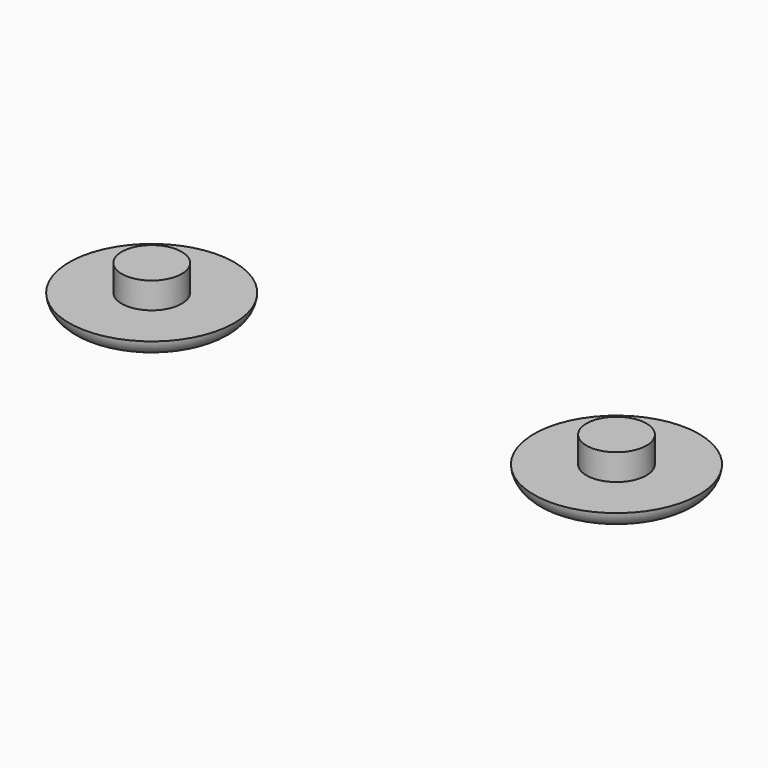
from build123d import *

# Parameters (mm, degrees)
F0_R     = 11
F1_DEPTH = 2.286
F2_R     = 4
F3_DEPTH = 3.5
F5_R     = 11
F6_DEPTH = 2.286
F7_R     = 4
F8_DEPTH = 3.5


# Not quite as in the source:
# - a fillet or chamfer that OpenCascade refuses, or shapes differently, is made with other operations: its cross-section is extruded or revolved along the edge and cut away or added


with BuildPart() as f1:
    # F0 (on Top) → F1 (new body)
    with BuildSketch(Plane.XY):
        Circle(F0_R)
    extrude(amount=F1_DEPTH)

    # F2 (on face) → F3 (join)
    with BuildSketch(Plane.XY.offset(2.286)):
        Circle(F2_R)
    extrude(amount=F3_DEPTH)

    # F4: fillet of radius 2.54 on 1 edges, made by hand

    # F4_s1 → F4_t2 (revolve, cut)
    with BuildSketch(Plane.XZ):
        with BuildLine():
            ThreePointArc((11, 2.286), (10.1766157086, 0.6562855843), (8.4727319097, 0))
            Line((8.4727319097, 0), (11, 0))
            Line((11, 0), (11, 2.286))
        make_face()
    revolve(axis=Axis((0, 0, 0), (0, 0, 1)), mode=Mode.SUBTRACT)


with BuildPart() as f6:
    # F5 (on Top) → F6 (new body)
    with BuildSketch(Plane.XY):
        with Locations((61.9736175734, 0)):
            Circle(F5_R)
    extrude(amount=F6_DEPTH)

    # F7 (on face) → F8 (join)
    with BuildSketch(Plane.XY.offset(2.286)):
        with Locations((61.9736175734, 0)):
            Circle(F7_R)
    extrude(amount=F8_DEPTH)

    # F9: fillet of radius 2.54 on 1 edges, made by hand

    # F9_s1 → F9_t2 (revolve, cut)
    with BuildSketch(Plane.XZ):
        with BuildLine():
            ThreePointArc((72.9736175734, 2.286), (72.150233282, 0.6562855843), (70.4463494832, 0))
            Line((70.4463494832, 0), (72.9736175734, 0))
            Line((72.9736175734, 0), (72.9736175734, 2.286))
        make_face()
    revolve(axis=Axis((61.9736175734, 0, 0), (0, 0, 1)), mode=Mode.SUBTRACT)


solid = Compound([f1.part, f6.part])
